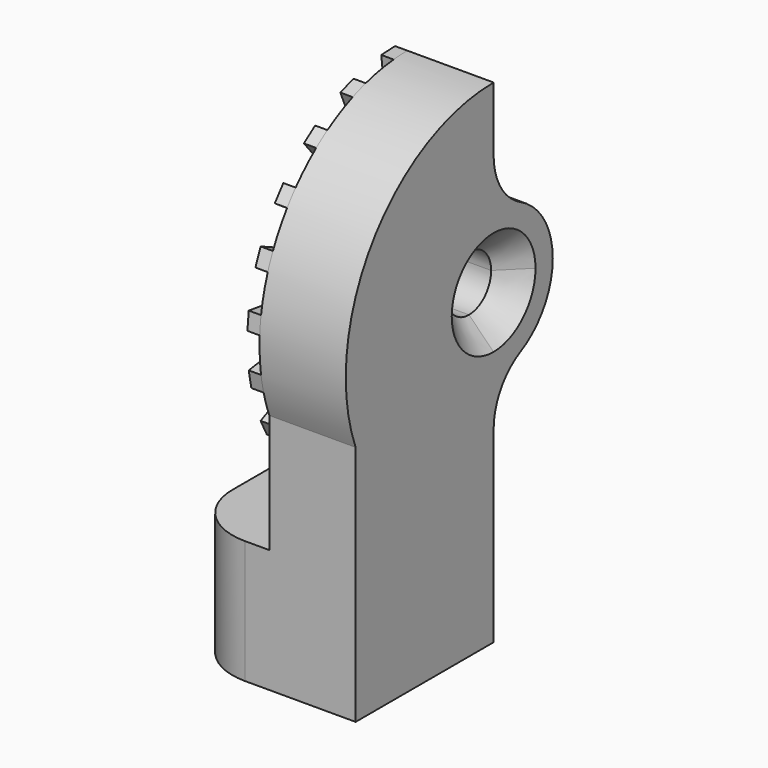
from build123d import *

# Parameters (mm, degrees)
F0_W         = 14
F0_H         = 14
F0_R         = 3
F1_DEPTH     = 10
F3_DEPTH     = 7
F5_DEPTH     = 1
F6_T1_DEPTH  = 7
F6_T6_DEPTH  = 7
F6_S7_R      = 6.75
F6_T8_DEPTH  = 6
F6_T12_DEPTH = 7
F6_S13_R     = 6.75
F6_T14_DEPTH = 6
F6_T18_DEPTH = 16.4948974278
F6_S20_R     = 6.75
F6_T21_DEPTH = 10
F7_R         = 5
F8_SIZE      = 2


# Not quite as in the source:
# - a fillet or chamfer that OpenCascade refuses, or shapes differently, is made with other operations: its cross-section is extruded or revolved along the edge and cut away or added


with BuildPart() as f1:
    # F0 (on Top) → F1 (new body)
    with BuildSketch(Plane.XY):
        Rectangle(F0_W, F0_H)
        Circle(F0_R, mode=Mode.SUBTRACT)
    extrude(amount=F1_DEPTH)

    # F2 (on face) → F3 (join)
    with BuildSketch(Plane.YZ.offset(7)):
        with BuildLine():
            Line((7, 31), (7, 40))
            ThreePointArc((7, 40), (-5.3648184804, 33.4918351342), (-7, 19.6148351929))
            ThreePointArc((-7, 19.6148351929), (-1.4918351342, 12.6351815196), (7, 10))
            Line((7, 10), (7, 19))
            Line((7, 19), (7, 22.75))
            ThreePointArc((7, 22.75), (4.75, 25), (7, 27.25))
            Line((7, 27.25), (7, 31))
        make_face()
        with BuildLine():
            ThreePointArc((7, 19), (13, 25), (7, 31))
            Line((7, 31), (7, 27.25))
            ThreePointArc((7, 27.25), (8.5909902577, 26.5909902577), (9.25, 25))
            ThreePointArc((9.25, 25), (8.5909902577, 23.4090097423), (7, 22.75))
            Line((7, 22.75), (7, 19))
        make_face()
        with BuildLine():
            ThreePointArc((7, 10), (-1.4918351342, 12.6351815196), (-7, 19.6148351929))
            Line((-7, 19.6148351929), (-7, 10))
            Line((-7, 10), (7, 10))
        make_face()
    extrude(amount=-F3_DEPTH)

    # F4 (on face) → F5 (join)
    with BuildSketch(Plane(origin=(0, 0, 0), x_dir=(0, -1, 0), z_dir=(-1, 0, 0))):
        with BuildLine():
            Line((-5.6015252753, 39.9346666667), (-7, 40))
            Line((-7, 40), (-7, 31.75))
            ThreePointArc((-7, 31.75), (-6.7748747563, 31.7462447795), (-6.55, 31.7349832962))
            Line((-6.55, 31.7349832962), (-5.6015252753, 39.9346666667))
        make_face()
        with BuildLine():
            Line((-1.4505915023, 38.9357118701), (-2.7740116474, 39.3923946042))
            Line((-2.7740116474, 39.3923946042), (-5.0983052413, 31.4765775719))
            ThreePointArc((-5.0983052413, 31.4765775719), (-4.8833571197, 31.4095493537), (-4.6707640976, 31.3353894995))
            Line((-4.6707640976, 31.3353894995), (-1.4505915023, 38.9357118701))
        make_face()
        with BuildLine():
            Line((2.2507621978, 36.8077685766), (1.1096122618, 37.6188029925))
            Line((1.1096122618, 37.6188029925), (-3.3506744822, 30.6784613466))
            ThreePointArc((-3.3506744822, 30.6784613466), (-3.1633173011, 30.5535903583), (-2.9802290354, 30.4225401236))
            Line((-2.9802290354, 30.4225401236), (2.2507621978, 36.8077685766))
        make_face()
        with BuildLine():
            Line((5.2026741611, 33.7232300966), (4.3362436153, 34.8229110092))
            Line((4.3362436153, 34.8229110092), (-1.8986903731, 29.4203099541))
            ThreePointArc((-1.8986903731, 29.4203099541), (-1.7541026971, 29.2477125006), (-1.6153519103, 29.070388796))
            Line((-1.6153519103, 29.070388796), (5.2026741611, 33.7232300966))
        make_face()
        with BuildLine():
            Line((7.1659980359, 29.9319873933), (6.6444799303, 31.231225195))
            Line((6.6444799303, 31.231225195), (-0.8599840314, 27.8040513378))
            ThreePointArc((-0.8599840314, 27.8040513378), (-0.7698794941, 27.5977102382), (-0.6867069498, 27.3884787756))
            Line((-0.6867069498, 27.3884787756), (7.1659980359, 29.9319873933))
        make_face()
        with BuildLine():
            Line((7.9816769983, 25.7411844029), (7.8473216282, 27.1347225741))
            Line((7.8473216282, 27.1347225741), (-0.3187052673, 25.9606251583))
            ThreePointArc((-0.3187052673, 25.9606251583), (-0.2903836024, 25.7372569414), (-0.2695274455, 25.5130684097))
            Line((-0.2695274455, 25.5130684097), (7.9816769983, 25.7411844029))
        make_face()
        with BuildLine():
            Line((-0.3976107999, 23.5960922926), (7.5836295897, 21.4903350603))
            Line((7.5836295897, 21.4903350603), (7.8473216282, 22.8652774259))
            Line((7.8473216282, 22.8652774259), (-0.3187052673, 24.0393748417))
            ThreePointArc((-0.3187052673, 24.0393748417), (-0.3544609277, 23.8170754719), (-0.3976107999, 23.5960922926))
        make_face()
        with BuildLine():
            ThreePointArc((-0.8599840314, 22.1959486622), (-0.9569203061, 21.9927275126), (-1.0605804615, 21.7928524285))
            Line((-1.0605804615, 21.7928524285), (6.004103244, 17.5238178982))
            Line((6.004103244, 17.5238178982), (6.6444799303, 18.768774805))
            Line((6.6444799303, 18.768774805), (-0.8599840314, 22.1959486622))
        make_face()
        with BuildLine():
            ThreePointArc((-1.8986903731, 20.5796900459), (-2.0489540617, 20.4120108852), (-2.2047265709, 20.2494365871))
            Line((-2.2047265709, 20.2494365871), (3.3710617919, 14.1629765475))
            Line((3.3710617919, 14.1629765475), (4.3362436153, 15.1770889908))
            Line((4.3362436153, 15.1770889908), (-1.8986903731, 20.5796900459))
        make_face()
        with BuildLine():
            ThreePointArc((-3.3506744822, 19.3215386534), (-3.5420921143, 19.2029858501), (-3.737357215, 19.0908831407))
            Line((-3.737357215, 19.0908831407), (-0.1021814076, 11.6800863867))
            Line((-0.1021814076, 11.6800863867), (1.1096122618, 12.3811970075))
            Line((1.1096122618, 12.3811970075), (-3.3506744822, 19.3215386534))
        make_face()
        with BuildLine():
            ThreePointArc((-5.0983052413, 18.5234224281), (-5.3153692987, 18.4636004253), (-5.5343077738, 18.4110511993))
            Line((-5.5343077738, 18.4110511993), (-4.1342448465, 10.2762964102))
            Line((-4.1342448465, 10.2762964102), (-2.7740116474, 10.6076053958))
            Line((-2.7740116474, 10.6076053958), (-5.0983052413, 18.5234224281))
        make_face()
    extrude(amount=F5_DEPTH)

    # F6: fillet of radius 5 on 2 edges, made by hand

    # F6_s2 → F6_t1 (join)
    with BuildSketch(Plane.YZ):
        with BuildLine():
            ThreePointArc((7, 15.2020410289), (7.7359856729, 17.8132058682), (9.7272727273, 19.655658743))
            ThreePointArc((9.7272727273, 19.655658743), (8.4024892973, 19.1662170274), (7, 19))
            Line((7, 19), (7, 15.2020410289))
        make_face()
    extrude(amount=F6_T1_DEPTH)


with BuildPart() as f6_tool4:
    # F6_s5 → F6_t6 (new body)
    with BuildSketch(Plane.YZ.offset(7)):
        with BuildLine():
            ThreePointArc((7, 34.7979589711), (7.7359856729, 32.1867941318), (9.7272727273, 30.344341257))
            ThreePointArc((9.7272727273, 30.344341257), (8.4024892973, 30.8337829726), (7, 31))
            Line((7, 31), (7, 34.7979589711))
        make_face()
    extrude(amount=-F6_T6_DEPTH)

    # F6_s7 → F6_t8 (cut, symmetric)
    with BuildSketch(Plane.YZ.offset(3.5)):
        with Locations((7, 25)):
            Circle(F6_S7_R)
    extrude(amount=F6_T8_DEPTH, both=True, mode=Mode.SUBTRACT)


with BuildPart() as f1_1:
    add(f1.part)

    # F6_t3: union F6_tool4
    add(f6_tool4.part)


with BuildPart() as f6_tool10:
    # F6_s11 → F6_t12 (new body)
    with BuildSketch(Plane.YZ.offset(7)):
        with BuildLine():
            ThreePointArc((7, 34.7979589711), (7.7359856729, 32.1867941318), (9.7272727273, 30.344341257))
            ThreePointArc((9.7272727273, 30.344341257), (8.4024892973, 30.8337829726), (7, 31))
            Line((7, 31), (7, 34.7979589711))
        make_face()
    extrude(amount=-F6_T12_DEPTH)

    # F6_s13 → F6_t14 (intersect, symmetric)
    with BuildSketch(Plane.YZ.offset(3.5)):
        with Locations((7, 25)):
            Circle(F6_S13_R)
    extrude(amount=F6_T14_DEPTH, both=True, mode=Mode.INTERSECT)


with BuildPart() as f1_2:
    add(f1_1.part)

    # F6_t9: union F6_tool10
    add(f6_tool10.part)


with BuildPart() as f6_tool16:
    # F6_s17 → F6_t18 (new body)
    with BuildSketch(Plane.YZ.offset(7)):
        with BuildLine():
            ThreePointArc((7, 34.7979589711), (7.7359856729, 32.1867941318), (9.7272727273, 30.344341257))
            ThreePointArc((9.7272727273, 30.344341257), (8.4024892973, 30.8337829726), (7, 31))
            Line((7, 31), (7, 34.7979589711))
        make_face()
    extrude(amount=-F6_T18_DEPTH)

    split(bisect_by=Plane.YZ, keep=Keep.BOTTOM)

    # F6_s20 → F6_t21 (cut, symmetric)
    with BuildSketch(Plane.YZ.offset(-1.2)):
        with Locations((7, 25)):
            Circle(F6_S20_R)
    extrude(amount=F6_T21_DEPTH, both=True, mode=Mode.SUBTRACT)

    split(bisect_by=Plane.YZ.offset(-1), keep=Keep.TOP)


with BuildPart() as f1_3:
    add(f1_2.part)

    # F6_t15: union F6_tool16
    add(f6_tool16.part)

    # F7
    f7_edges = [f1_3.edges().sort_by_distance(p)[0] for p in [
        (-7, 7, 5),
        (-7, -7, 5),
    ]]
    fillet(f7_edges, radius=F7_R)

    # F8
    f8_edges = [f1_3.edges().sort_by_distance(p)[0] for p in [
        (7, 7, 22.75),
    ]]
    chamfer(f8_edges, length=F8_SIZE)


solid = f1_3.part
